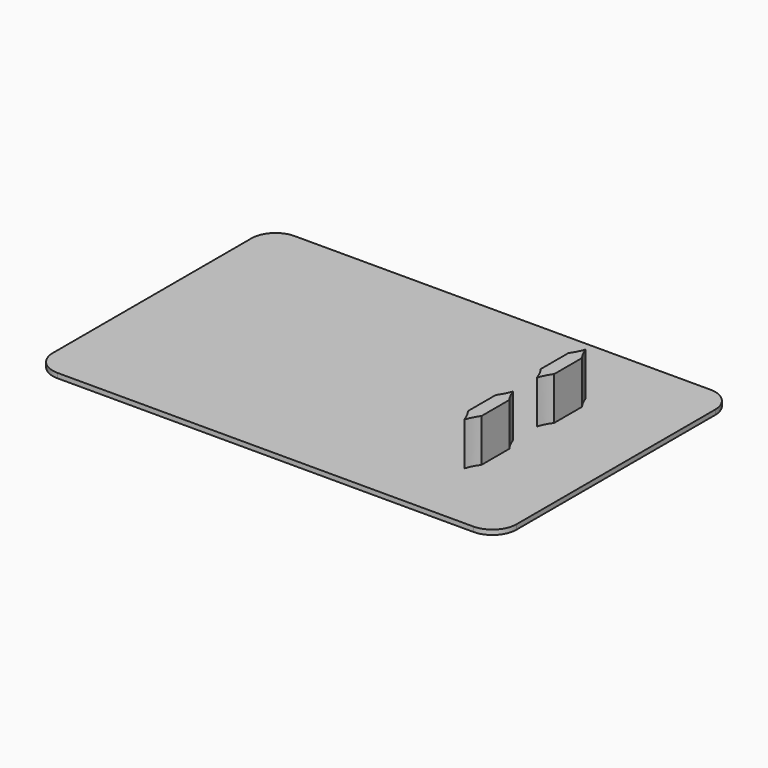
from build123d import *

# Parameters (mm, degrees)
F0_W     = 59
F0_H     = 62
F0_W_2   = 38
F1_DEPTH = 1
F2_DEPTH = 10
F3_R     = 5


# Not quite as in the source:
# - a feature names something its author has since deleted; it is built from what else it names


with BuildPart() as f1:
    # F0 (on Top) → F1 (new body)
    with BuildSketch(Plane.XY):
        with Locations((-39, 19)):
            Rectangle(F0_W, F0_H)
        with Locations((9.5, 19)):
            Rectangle(F0_W_2, F0_H)
        with BuildLine():
            ThreePointArc((9.5, 15.8775010008), (10.0985618966, 14.4432029131), (10.9121369044, 13.1189736826))
            Line((10.9121369044, 13.1189736826), (10.9121369044, 5.8810263174))
            ThreePointArc((10.9121369044, 5.8810263174), (10.0985618966, 4.5567970869), (9.5, 3.1224989992))
            ThreePointArc((9.5, 3.1224989992), (8.9014381034, 4.5567970869), (8.0878630956, 5.8810263174))
            Line((8.0878630956, 5.8810263174), (8.0878630956, 13.1189736826))
            ThreePointArc((8.0878630956, 13.1189736826), (8.9014381034, 14.4432029131), (9.5, 15.8775010008))
        make_face(mode=Mode.SUBTRACT)
        with BuildLine():
            Line((8.0878630956, 24.8810263174), (8.0878630956, 32.1189736826))
            ThreePointArc((8.0878630956, 32.1189736826), (8.9014381034, 33.4432029131), (9.5, 34.8775010008))
            ThreePointArc((9.5, 34.8775010008), (10.0985618966, 33.4432029131), (10.9121369044, 32.1189736826))
            Line((10.9121369044, 32.1189736826), (10.9121369044, 24.8810263174))
            ThreePointArc((10.9121369044, 24.8810263174), (10.0985618966, 23.5567970869), (9.5, 22.1224989992))
            ThreePointArc((9.5, 22.1224989992), (8.9014381034, 23.5567970869), (8.0878630956, 24.8810263174))
        make_face(mode=Mode.SUBTRACT)
    extrude(amount=F1_DEPTH)

    # F0 (on Top) → F2 (join)
    with BuildSketch(Plane.XY):
        with BuildLine():
            ThreePointArc((9.5, 34.8775010008), (8.9014381034, 33.4432029131), (8.0878630956, 32.1189736826))
            Line((8.0878630956, 32.1189736826), (8.0878630956, 24.8810263174))
            ThreePointArc((8.0878630956, 24.8810263174), (8.9014381034, 23.5567970869), (9.5, 22.1224989992))
            ThreePointArc((9.5, 22.1224989992), (10.0985618966, 23.5567970869), (10.9121369044, 24.8810263174))
            Line((10.9121369044, 24.8810263174), (10.9121369044, 32.1189736826))
            ThreePointArc((10.9121369044, 32.1189736826), (10.0985618966, 33.4432029131), (9.5, 34.8775010008))
        make_face()
        with BuildLine():
            Line((10.9121369044, 5.8810263174), (10.9121369044, 13.1189736826))
            ThreePointArc((10.9121369044, 13.1189736826), (10.0985618966, 14.4432029131), (9.5, 15.8775010008))
            ThreePointArc((9.5, 15.8775010008), (8.9014381034, 14.4432029131), (8.0878630956, 13.1189736826))
            Line((8.0878630956, 13.1189736826), (8.0878630956, 5.8810263174))
            ThreePointArc((8.0878630956, 5.8810263174), (8.9014381034, 4.5567970869), (9.5, 3.1224989992))
            ThreePointArc((9.5, 3.1224989992), (10.0985618966, 4.5567970869), (10.9121369044, 5.8810263174))
        make_face()
    extrude(amount=F2_DEPTH)

    # F3
    f3_edges = [f1.edges().sort_by_distance(p)[0] for p in [
        (-68.5, 50, 0.5),
        (28.5, 50, 0.5),
        (28.5, -12, 0.5),
        (-68.5, -12, 0.5),
    ]]
    fillet(f3_edges, radius=F3_R)


solid = f1.part
